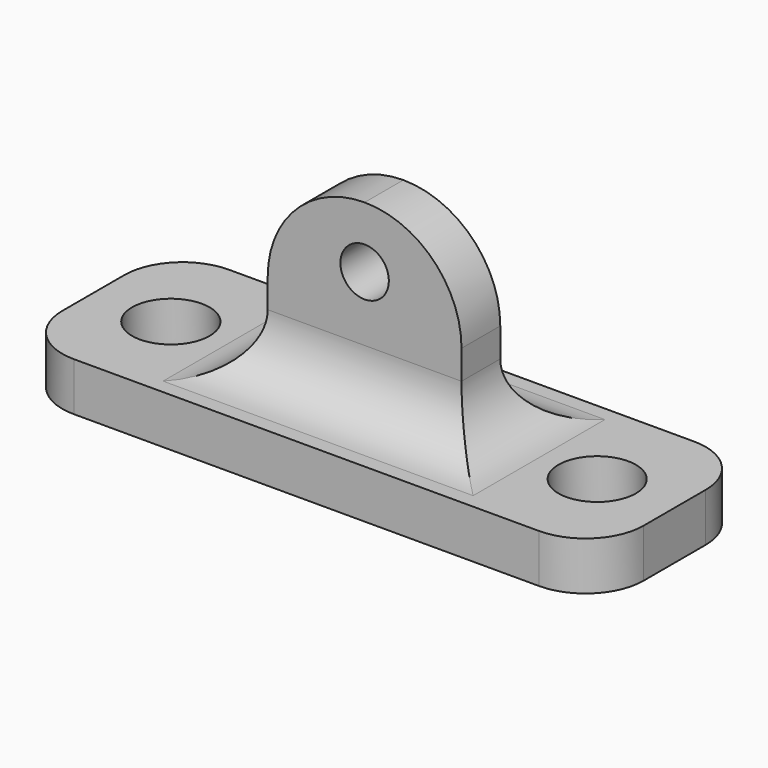
from build123d import *

# Parameters (mm, degrees)
F0_W     = 38.1
F0_H     = 12.7
F0_W_2   = 12.7
F0_H_2   = 3.175
F1_DEPTH = 3.175
F2_DEPTH = 15.24
F3_R     = 6.34999
F4_R     = 3.81
F5_R     = 1.5875
F6_DEPTH = 12.701
F7_R     = 2.54
F8_DEPTH = 3.176


# Not quite as in the source:
# - a fillet or chamfer is up to 0.001 mm smaller than in the source, because OpenCascade refuses the exact size


with BuildPart() as f1:
    # F0 (on Top) → F1 (new body)
    with BuildSketch(Plane.XY):
        Rectangle(F0_W, F0_H)
        Rectangle(F0_W_2, F0_H_2, mode=Mode.SUBTRACT)
    extrude(amount=F1_DEPTH)

    # F0 (on Top) → F2 (join)
    with BuildSketch(Plane.XY):
        Rectangle(F0_W_2, F0_H_2)
    extrude(amount=F2_DEPTH)

    # F3 (radius 6.35 in the source; OpenCascade refuses exactly that, so slightly less here)
    f3_edges = [f1.edges().sort_by_distance(p)[0] for p in [
        (-6.35, 0, 15.24),
        (6.35, 0, 15.24),
    ]]
    fillet(f3_edges, radius=F3_R)

    # F4 (call 1 of 5: OpenCascade refuses the feature's edges together)
    f4_edges = [f1.edges().sort_by_distance(p)[0] for p in [
        (-19.05, -6.35, 1.5875),
    ]]
    fillet(f4_edges, radius=F4_R)

    # F4#2 (call 2 of 5)
    f4_2_edges = [f1.edges().sort_by_distance(p)[0] for p in [
        (-19.05, 6.35, 1.5875),
    ]]
    fillet(f4_2_edges, radius=F4_R)

    # F4#3 (call 3 of 5)
    f4_3_edges = [f1.edges().sort_by_distance(p)[0] for p in [
        (19.05, 6.35, 1.5875),
    ]]
    fillet(f4_3_edges, radius=F4_R)

    # F4#4 (call 4 of 5)
    f4_4_edges = [f1.edges().sort_by_distance(p)[0] for p in [
        (19.05, -6.35, 1.5875),
    ]]
    fillet(f4_4_edges, radius=F4_R)

    # F4#5 (call 5 of 5)
    f4_5_edges = [f1.edges().sort_by_distance(p)[0] for p in [
        (0, -1.5875, 3.175),
        (0, 1.5875, 3.175),
        (6.35, 0, 3.175),
        (-6.35, 0, 3.175),
    ]]
    fillet(f4_5_edges, radius=F4_R)

    # F5 (on face) → F6 (cut, through all)
    with BuildSketch(Plane.XZ.offset(6.35)):
        with Locations((0, 11.2299183384)):
            Circle(F5_R)
    extrude(amount=-F6_DEPTH, mode=Mode.SUBTRACT)

    # F7 (on face) → F8 (cut, through all)
    with BuildSketch(Plane.XY.offset(3.175)):
        with Locations((-13.97, 0)):
            Circle(F7_R)
        with Locations((13.97, 0)):
            Circle(F7_R)
    extrude(amount=-F8_DEPTH, mode=Mode.SUBTRACT)


solid = f1.part
